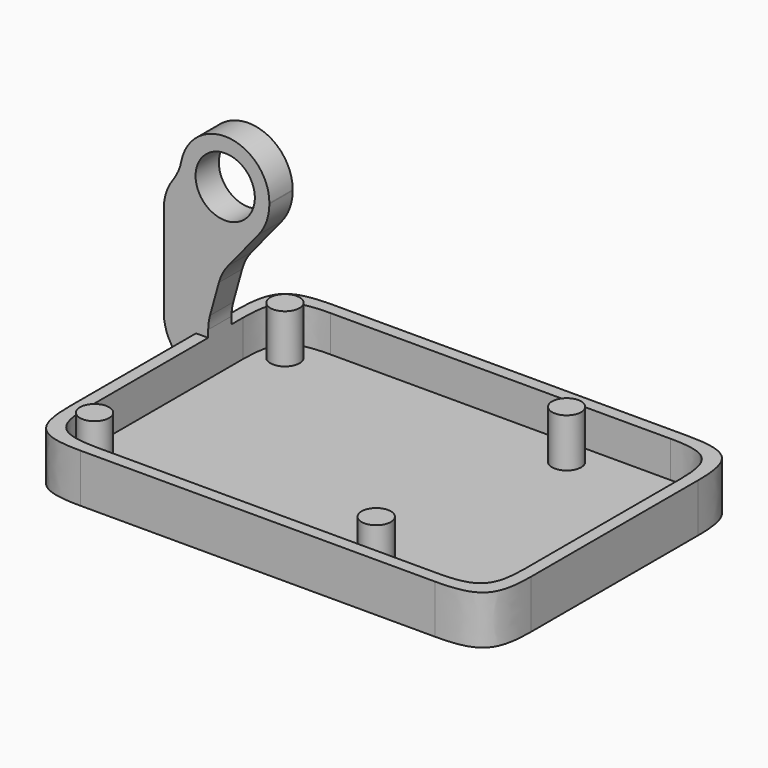
from build123d import *

# Parameters (mm, degrees)
F0_W        = 90
F0_H        = 60
F1_DEPTH    = 2.5
F2_W        = 95
F2_H        = 65
F2_W_2      = 90
F2_H_2      = 60
F3_DEPTH    = 10
F4_T1_DEPTH = 7.5
F5_T1_DEPTH = 65
F6_R        = 3
F7_DEPTH    = 10
F10_R       = 6.1
F11_DEPTH   = 6
F12_R       = 10


# Not quite as in the source:
# - a fillet or chamfer that OpenCascade refuses, or shapes differently, is made with other operations: its cross-section is extruded or revolved along the edge and cut away or added


with BuildPart() as f1:
    # F0 (on Top) → F1 (new body)
    with BuildSketch(Plane.XY):
        Rectangle(F0_W, F0_H)
    extrude(amount=F1_DEPTH)

    # F2 (on Top) → F3 (join)
    with BuildSketch(Plane.XY):
        Rectangle(F2_W, F2_H)
        Rectangle(F2_W_2, F2_H_2, mode=Mode.SUBTRACT)
    extrude(amount=F3_DEPTH)

    # F4: fillet of radius 10 on 4 edges, made by hand

    # F4_s2 → F4_t1 (join)
    with BuildSketch(Plane.XY.offset(2.5)):
        with BuildLine():
            add(Edge.make_bspline(
                [(-45, 20), (-45, 30), (-35, 30)],
                knots=[0, 0, 0, 1, 1, 1], degree=2, weights=[1, 1.5, 1]))
            Line((-35, 30), (-45, 30))
            Line((-45, 30), (-45, 20))
        make_face()
        with BuildLine():
            add(Edge.make_bspline(
                [(45, 20), (45, 30), (35, 30)],
                knots=[0, 0, 0, 1, 1, 1], degree=2, weights=[1, 1.5, 1]))
            Line((35, 30), (45, 30))
            Line((45, 30), (45, 20))
        make_face()
        with BuildLine():
            add(Edge.make_bspline(
                [(45, -20), (45, -30), (35, -30)],
                knots=[0, 0, 0, 1, 1, 1], degree=2, weights=[1, 1.5, 1]))
            Line((35, -30), (45, -30))
            Line((45, -30), (45, -20))
        make_face()
        with BuildLine():
            add(Edge.make_bspline(
                [(-35, -30), (-45, -30), (-45, -20)],
                knots=[0, 0, 0, 1, 1, 1], degree=2, weights=[1, 1.5, 1]))
            Line((-45, -20), (-45, -30))
            Line((-45, -30), (-35, -30))
        make_face()
    extrude(amount=F4_T1_DEPTH)

    # F5: fillet of radius 11 on 4 edges, made by hand

    # F5_s2 → F5_t1 (cut)
    with BuildSketch(Plane.XY.offset(-27.5)):
        with BuildLine():
            add(Edge.make_bspline(
                [(-36.5, 32.5), (-47.5, 32.5), (-47.5, 21.5)],
                knots=[0, 0, 0, 1, 1, 1], degree=2, weights=[1, 1.5, 1]))
            Line((-47.5, 21.5), (-47.5, 32.5))
            Line((-47.5, 32.5), (-36.5, 32.5))
        make_face()
        with BuildLine():
            add(Edge.make_bspline(
                [(-36.5, -32.5), (-47.5, -32.5), (-47.5, -21.5)],
                knots=[0, 0, 0, 1, 1, 1], degree=2, weights=[1, 1.5, 1]))
            Line((-47.5, -21.5), (-47.5, -32.5))
            Line((-47.5, -32.5), (-36.5, -32.5))
        make_face()
        with BuildLine():
            add(Edge.make_bspline(
                [(47.5, 21.5), (47.5, 32.5), (36.5, 32.5)],
                knots=[0, 0, 0, 1, 1, 1], degree=2, weights=[1, 1.5, 1]))
            Line((36.5, 32.5), (47.5, 32.5))
            Line((47.5, 32.5), (47.5, 21.5))
        make_face()
        with BuildLine():
            add(Edge.make_bspline(
                [(36.5, -32.5), (47.5, -32.5), (47.5, -21.5)],
                knots=[0, 0, 0, 1, 1, 1], degree=2, weights=[1, 1.5, 1]))
            Line((47.5, -21.5), (47.5, -32.5))
            Line((47.5, -32.5), (36.5, -32.5))
        make_face()
    extrude(amount=F5_T1_DEPTH, mode=Mode.SUBTRACT)

    # F6 (on face) → F7 (join)
    with BuildSketch(Plane.XY.offset(2.5)):
        with Locations((-40, 24.5)):
            Circle(F6_R)
        with Locations((-40, -24.5)):
            Circle(F6_R)
        with Locations((18, -24.5)):
            Circle(F6_R)
        with Locations((18, 24.5)):
            Circle(F6_R)
    extrude(amount=F7_DEPTH)

    # F10 (on offset) → F11 (join)
    with BuildSketch(Plane(origin=(0, 11, 0), x_dir=(-1, 0, 0), z_dir=(0, 1, 0))):
        with BuildLine():
            Line((45, 0), (47.5, 0))
            Line((47.5, 0), (54.148522424, 8.0868878322))
            Line((54.148522424, 8.0868878322), (54.148522424, 33.5947699827))
            Line((54.148522424, 33.5947699827), (50.6855217688, 38.5))
            ThreePointArc((50.6855217688, 38.5), (41.5427608844, 47.6427608844), (32.4, 38.5))
            Line((32.4, 38.5), (32.4, 34.8039232194))
            Line((32.4, 34.8039232194), (42.2389033973, 22.7499233782))
            Line((42.2389033973, 22.7499233782), (45, 12.8317605704))
            Line((45, 12.8317605704), (45, 0))
        make_face()
        with Locations((41.5, 38.5)):
            Circle(F10_R, mode=Mode.SUBTRACT)
    extrude(amount=F11_DEPTH)

    # F12
    f12_edges = [f1.edges().sort_by_distance(p)[0] for p in [
        (-32.4, 14, 34.803923),
        (-42.238903, 14, 22.749923),
        (-45, 14, 12.831761),
        (-50.685522, 14, 38.5),
        (-54.148522, 14, 33.59477),
        (-54.148522, 14, 8.086888),
    ]]
    fillet(f12_edges, radius=F12_R)


solid = f1.part
